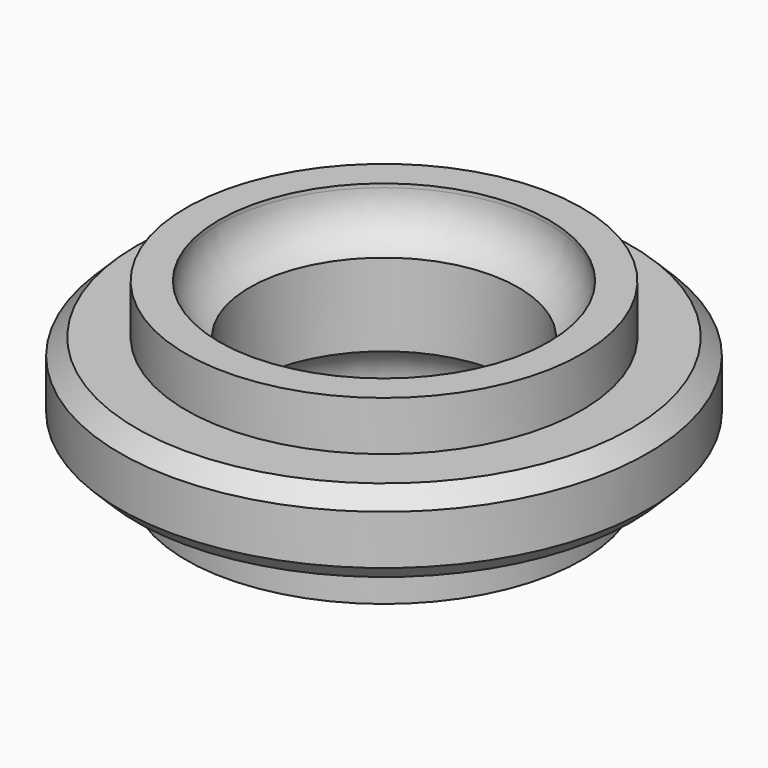
from build123d import *

# Parameters (mm, degrees)
F0_W    = 1.85
F0_H    = 5
F3_SIZE = 1


# Not quite as in the source:
# - a fillet or chamfer that OpenCascade refuses, or shapes differently, is made with other operations: its cross-section is extruded or revolved along the edge and cut away or added


with BuildPart() as f1:
    # F0 (on Right) → F1 (revolve)
    with BuildSketch(Plane.YZ):
        with Locations((1.6295755848, 1.9221331838)):
            Rectangle(F0_W, F0_H)
        Polygon((2.5545755848, 7.4221331838), (2.5545755848, 4.4221331838), (2.5545755848, -0.5778668162), (2.5545755848, -3.5778668162), (4.5545755848, -3.5778668162), (4.5545755848, -0.5778668162), (8.5545755848, -0.5778668162), (8.5545755848, 4.4221331838), (4.5545755848, 4.4221331838), (4.5545755848, 7.4221331838), align=None)
    revolve(axis=Axis((0, -7.4454244152, 1.9221331838), (0, 0, -1)))

    # F2: fillet of radius 3 on 2 edges, made by hand

    # F2_s1 → F2_t2 (revolve)
    with BuildSketch(Plane.YZ):
        with BuildLine():
            ThreePointArc((0.7045755848, 4.4221331838), (2.0495705748, 5.5271302594), (2.5545755848, 7.1929633843))
            Line((2.5545755848, 7.1929633843), (2.5545755848, 4.4221331838))
            Line((2.5545755848, 4.4221331838), (0.7045755848, 4.4221331838))
        make_face()
    revolve(axis=Axis((0, -7.4454244152, 4.4221331838), (0, 0, -1)))

    # F2_s3 → F2_t4 (revolve)
    with BuildSketch(Plane.YZ):
        with BuildLine():
            ThreePointArc((0.7045755848, -0.5778668162), (2.0495705748, -1.6828638918), (2.5545755848, -3.3486970167))
            Line((2.5545755848, -3.3486970167), (2.5545755848, -0.5778668162))
            Line((2.5545755848, -0.5778668162), (0.7045755848, -0.5778668162))
        make_face()
    revolve(axis=Axis((0, -7.4454244152, -0.5778668162), (0, 0, -1)))

    # F3
    f3_edges = [f1.edges().sort_by_distance(p)[0] for p in [
        (0, -23.445424, -0.577867),
        (0, -23.445424, 4.422133),
    ]]
    chamfer(f3_edges, length=F3_SIZE)


solid = f1.part
